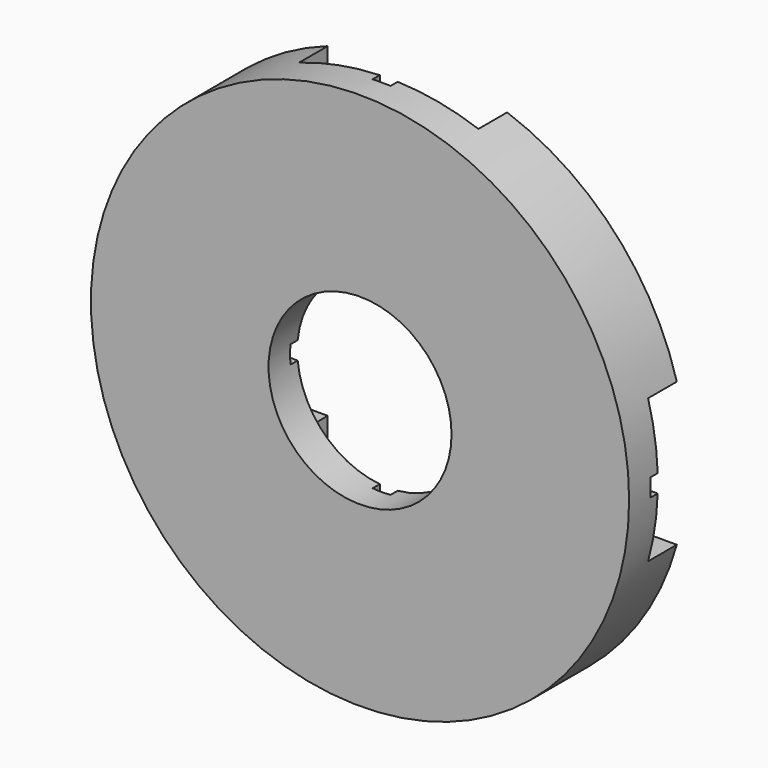
from build123d import *

# Parameters (mm, degrees)
F0_R          = 12.7
F1_DEPTH      = 17.78
F2_R          = 38.1
F3_DEPTH      = 10.16
F4_R          = 12.954
F5_DEPTH      = 17.781
F5_DEPTH_BACK = 115
F6_W          = 5.08
F6_H          = 20.32
F7_DEPTH      = 38.101
F7_DEPTH_BACK = 38.101
F8_W          = 25.4
F8_H          = 5.08
F9_DEPTH      = 38.101
F9_DEPTH_BACK = 38.101
F11_DEPTH     = 6.35


# Not quite as in the source:
# - an extrude ends at something that could not be found from the text; its depth is read off the source's solid


with BuildPart() as f1:
    # F0 (on Front) → F1 (new body)
    with BuildSketch(Plane.XZ):
        Circle(F0_R)
    extrude(amount=F1_DEPTH)

    # F2 (on Front) → F3 (join)
    with BuildSketch(Plane.XZ):
        Circle(F2_R)
    extrude(amount=F3_DEPTH)

    # F4 (on Front) → F5 (cut, two sides)
    with BuildSketch(Plane.XZ) as f5_sk:
        Circle(F4_R)
    extrude(amount=F5_DEPTH, mode=Mode.SUBTRACT)
    extrude(f5_sk.sketch, amount=-F5_DEPTH_BACK, mode=Mode.SUBTRACT)

    # F6 (on Right) → F7 (cut, two sides)
    with BuildSketch(Plane.YZ) as f7_sk:
        with Locations((-2.54, 0)):
            Rectangle(F6_W, F6_H)
    extrude(amount=F7_DEPTH, mode=Mode.SUBTRACT)
    extrude(f7_sk.sketch, amount=-F7_DEPTH_BACK, mode=Mode.SUBTRACT)

    # F8 (on Top) → F9 (cut, two sides)
    with BuildSketch(Plane.XY) as f9_sk:
        with Locations((0, -2.54)):
            Rectangle(F8_W, F8_H)
    extrude(amount=-F9_DEPTH, mode=Mode.SUBTRACT)
    extrude(f9_sk.sketch, amount=F9_DEPTH_BACK, mode=Mode.SUBTRACT)

    # F10 (on face) → F11 (cut)
    with BuildSketch(Plane(origin=(0, 0, 0), x_dir=(-1, 0, 0), z_dir=(0, 1, 0))):
        with BuildLine():
            Line((1.27, -1.27), (38.0788274504, -1.27))
            ThreePointArc((38.0788274504, -1.27), (38.1, 0), (38.0788274504, 1.27))
            Line((38.0788274504, 1.27), (1.27, 1.27))
            Line((1.27, 1.27), (1.27, 38.0788274504))
            ThreePointArc((1.27, 38.0788274504), (0, 38.1), (-1.27, 38.0788274504))
            Line((-1.27, 38.0788274504), (-1.27, 1.27))
            Line((-1.27, 1.27), (-38.0788274504, 1.27))
            ThreePointArc((-38.0788274504, 1.27), (-38.1, 0), (-38.0788274504, -1.27))
            Line((-38.0788274504, -1.27), (-1.27, -1.27))
            Line((-1.27, -1.27), (-1.27, -38.0788274504))
            ThreePointArc((-1.27, -38.0788274504), (0, -38.1), (1.27, -38.0788274504))
            Line((1.27, -38.0788274504), (1.27, -1.27))
        make_face()
    extrude(amount=-F11_DEPTH, mode=Mode.SUBTRACT)


solid = f1.part
